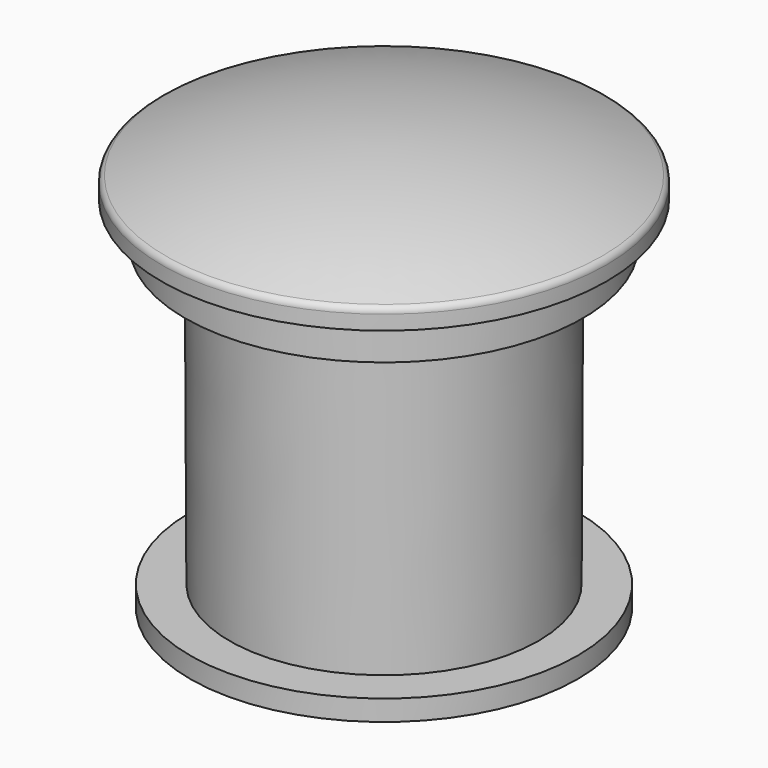
from build123d import *

# Parameters (mm, degrees)
F0_W = 4.7118738294
F0_H = 1.9611492753


# Not quite as in the source:
# - ends of sketch curves that miss each other by under 0.0002 mm in the source are joined


with BuildPart() as f1:
    # F0 (on Front) → F1 (revolve)
    with BuildSketch(Plane.XZ):
        with BuildLine():
            Line((-22.8879310345, -32.9238119473), (-21.2663058621, -32.9238119473))
            Line((-21.2663058621, -32.9238119473), (-21.0060344828, 25.4316028803))
            ThreePointArc((-21.0060344828, 25.4316028803), (-10.5161670114, 26.2200468641), (0, 26.4830846044))
            Line((0, 26.4830846044), (0, 31.9253259837))
            ThreePointArc((0, 31.9253259837), (-16.4971879997, 30.3737453745), (-32.4157818514, 25.7734210307))
            ThreePointArc((-32.4157818514, 25.7734210307), (-32.8839026766, 25.3994841562), (-33.0603448276, 24.8269139147))
            Line((-33.0603448276, 24.8269139147), (-33.0603448276, 22.668429432))
            Line((-33.0603448276, 22.668429432), (-29.5, 22.668429432))
            Line((-29.5, 22.668429432), (-29.5, 16.666705294))
            Line((-29.5, 16.666705294), (-25.075, 16.666705294))
            Line((-25.075, 16.666705294), (-25.075, 23.0670863285))
            Line((-25.075, 23.0670863285), (-25.075, 25.0425487423))
            ThreePointArc((-25.075, 25.0425487423), (-24.1096353651, 25.1413648367), (-23.142241947, 25.2178075116))
            Line((-23.142241947, 25.2178075116), (-22.9110770379, -27.6320762932))
            Line((-22.9110770379, -27.6320762932), (-28.7643186748, -27.6320762932))
            Line((-28.7643186748, -27.6320762932), (-28.7643186748, -30.6968204677))
            Line((-28.7643186748, -30.6968204677), (-22.8976718749, -30.6968204677))
            Line((-22.8976718749, -30.6968204677), (-22.8879310345, -32.9238119473))
        make_face()
        with Locations((-25.4785697907, -29.2394068092)):
            Rectangle(F0_W, F0_H, mode=Mode.SUBTRACT)
    revolve(axis=Axis((0, 0, -4.8374448988), (0, 0, -1)))


solid = f1.part
